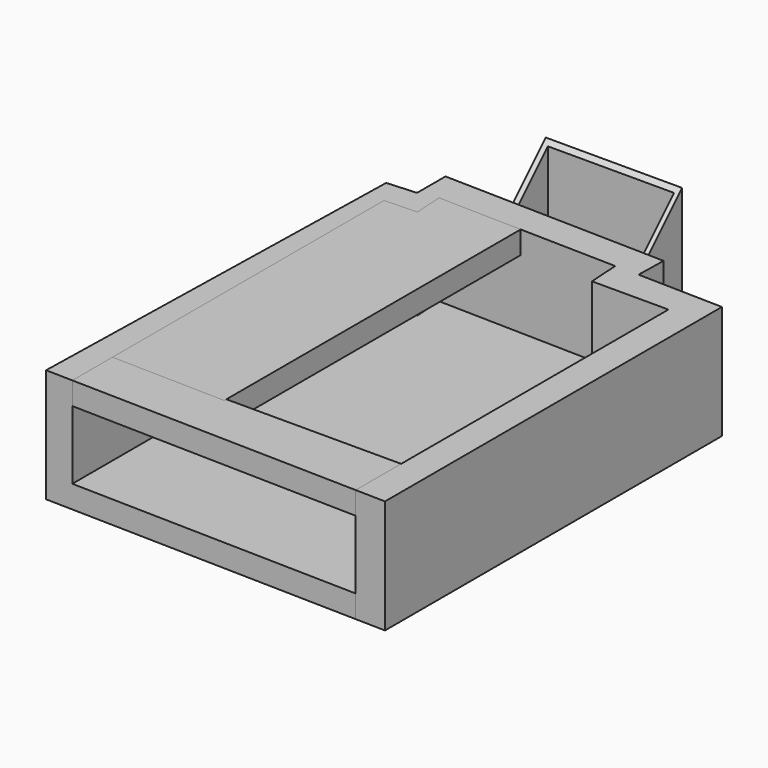
from build123d import *

# Parameters (mm, degrees)
F1_DEPTH     = 51.054
F2_DEPTH     = 10.16
F4_DEPTH     = 10.16
F6_DEPTH     = 10.16
F7_W         = 56.6421095282
F7_H         = 30.7425558567
F8_DEPTH     = 10.16
F7_W_2       = 61.2745471299
F7_H_2       = 34.6380155534
F9_DEPTH     = 63.5
F10_T1_DEPTH = 322.5575387072


# Not quite as in the source:
# - a fillet or chamfer that OpenCascade refuses, or shapes differently, is made with other operations: its cross-section is extruded or revolved along the edge and cut away or added


with BuildPart() as f1:
    # F0 (on Top) → F1 (new body)
    with BuildSketch(Plane.XY):
        Polygon((-35.2039023449, -49.0766943542), (-48.3769522073, -49.9528594767), (-52.6391126395, -235.6071644364), (-40.6254976988, -235.8829671131), (-40.6254976988, -60.8498267829), (-25.9644463658, -60.3935308754), (-26.8402741919, -47.2255522284), (53.7931299761, -49.0766943542), (54.7347292304, -63.2335394621), (89.056285343, -63.2335394621), (89.056285343, -238.8601378529), (102.4658605456, -239.1679883003), (102.4658605456, -49.9528594767), (64.3012185928, -49.0766943542), (64.6151083374, -35.4040550191), (-35.2039023449, -33.1124591533), align=None)
    extrude(amount=F1_DEPTH)

    # F0 (on Top) → F2 (join)
    with BuildSketch(Plane.XY):
        Polygon((-40.6254976988, -60.8498267829), (-40.6254976988, -235.8829671131), (89.056285343, -238.8601378529), (89.056285343, -63.2335394621), (54.7347292304, -63.2335394621), (53.7931299761, -49.0766943542), (-26.8402741919, -47.2255522284), (-25.9644463658, -60.3935308754), align=None)
    extrude(amount=F2_DEPTH)


with BuildPart() as f4:
    # F3 (on face) → F4 (new body)
    with BuildSketch(Plane.XY.offset(51.054)):
        Polygon((-40.6254976988, -213.3320122957), (-40.6254976988, -235.8829671131), (89.056285343, -238.8601378529), (89.056285343, -213.3320122957), align=None)
    extrude(amount=-F4_DEPTH)


with BuildPart() as f6:
    # F5 (on face) → F6 (new body)
    with BuildSketch(Plane.XY.offset(51.054)):
        Polygon((-40.6254976988, -60.8498267829), (-40.6254976988, -213.3318930864), (10.5520575639, -214.5068022872), (10.5520575639, -48.0839870323), (-26.8402741919, -47.2255522284), (-25.9644463658, -60.3935308754), align=None)
    extrude(amount=-F6_DEPTH)


with BuildPart() as f8:
    # F7 (on Top) → F8 (new body)
    with BuildSketch(Plane.XY):
        with Locations((0.1666704193, 0.2558268607)):
            Rectangle(F7_W, F7_H)
    extrude(amount=F8_DEPTH)

    # F7 (on Top) → F9 (join)
    with BuildSketch(Plane.XY):
        with Locations((-0.0438950956, 0.2031857148)):
            Rectangle(F7_W_2, F7_H_2)
        with Locations((0.1666704193, 0.2558268607)):
            Rectangle(F7_W, F7_H, mode=Mode.SUBTRACT)
    extrude(amount=F9_DEPTH)

    # F10: chamfer of 50.8 on 1 edges, made by hand

    # F10_s2 → F10_t1 (cut)
    with BuildSketch(Plane.YZ.offset(-161.3226644492)):
        Polygon((-17.1158220619, 12.7), (33.6841779381, 63.5), (-17.1158220619, 63.5), align=None)
    extrude(amount=F10_T1_DEPTH, mode=Mode.SUBTRACT)


solid = Compound([f1.part, f4.part, f6.part, f8.part])
